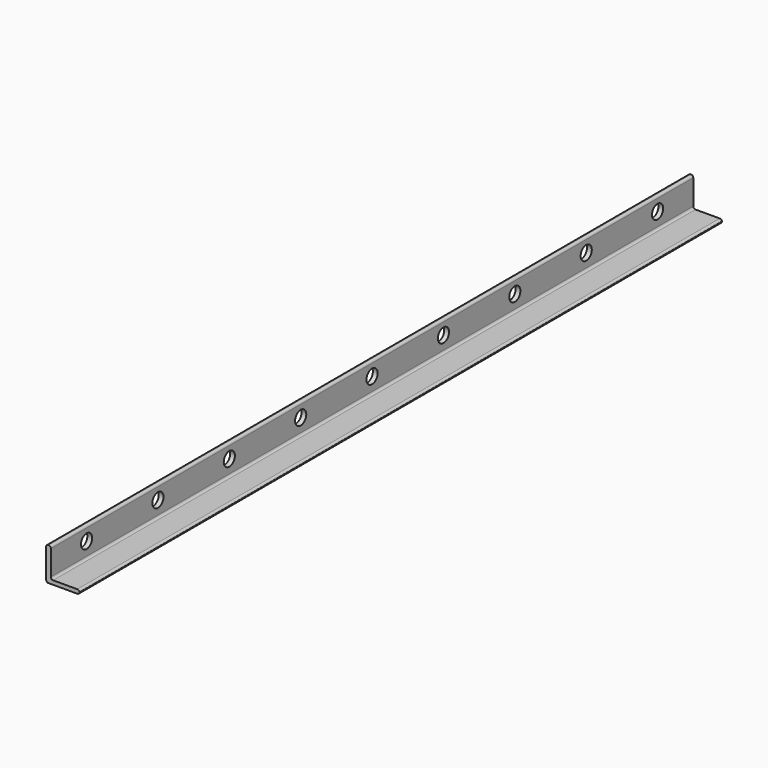
from build123d import *

# Parameters (mm, degrees)
F1_DEPTH    = 228.6
F3_D        = 7.9375
F4_T1_DEPTH = 457.2
F4_T3_DEPTH = 463.55


# Not quite as in the source:
# - a fillet or chamfer that OpenCascade refuses, or shapes differently, is made with other operations: its cross-section is extruded or revolved along the edge and cut away or added


with BuildPart() as f1:
    # F0 (on Front) → F1 (new body, symmetric)
    with BuildSketch(Plane.XZ):
        Polygon((0, 2.264165209), (0, 0), (2.7281190167, 0), (19.05, 0), (19.05, 2.264165209), (2.7281190167, 2.264165209), (2.7281190167, 19.05), (0, 19.05), align=None)
    extrude(amount=F1_DEPTH, both=True)

    # F3 (through all)
    with Locations(Plane.YZ.offset(2.7281190167)):
        with Locations((-203.2, 11.1125), (-152.4, 11.1125), (-101.6, 11.1125), (-50.8, 11.1125), (101.6, 11.1125), (50.8, 11.1125), (0, 11.1125), (152.4, 11.1125), (203.2, 11.1125)):
            Hole(F3_D / 2)

    # F4: fillet of radius 1.27 on 6 edges, made by hand

    # F4_s2 → F4_t1 (join)
    with BuildSketch(Plane.XZ.offset(-228.6)):
        with BuildLine():
            ThreePointArc((3.9981190167, 2.264165209), (3.1000934046, 2.6361395969), (2.7281190167, 3.534165209))
            Line((2.7281190167, 3.534165209), (2.7281190167, 2.264165209))
            Line((2.7281190167, 2.264165209), (3.9981190167, 2.264165209))
        make_face()
    extrude(amount=F4_T1_DEPTH)

    # F4_s4 → F4_t3 (cut)
    with BuildSketch(Plane.XZ.offset(-231.775)):
        with BuildLine():
            ThreePointArc((0, 17.78), (0.3719743879, 18.6780256121), (1.27, 19.05))
            Line((1.27, 19.05), (0, 19.05))
            Line((0, 19.05), (0, 17.78))
        make_face()
        with BuildLine():
            ThreePointArc((1.4581190167, 19.05), (2.3561446288, 18.6780256121), (2.7281190167, 17.78))
            Line((2.7281190167, 17.78), (2.7281190167, 19.05))
            Line((2.7281190167, 19.05), (1.4581190167, 19.05))
        make_face()
        with BuildLine():
            ThreePointArc((19.05, 0.994165209), (18.6780256121, 1.8921908211), (17.78, 2.264165209))
            Line((17.78, 2.264165209), (19.05, 2.264165209))
            Line((19.05, 2.264165209), (19.05, 0.994165209))
        make_face()
        with BuildLine():
            ThreePointArc((17.78, 0), (18.6780256121, 0.3719743879), (19.05, 1.27))
            Line((19.05, 1.27), (19.05, 0))
            Line((19.05, 0), (17.78, 0))
        make_face()
        with BuildLine():
            ThreePointArc((0, 1.27), (0.3719743879, 0.3719743879), (1.27, 0))
            Line((1.27, 0), (0, 0))
            Line((0, 0), (0, 1.27))
        make_face()
    extrude(amount=F4_T3_DEPTH, mode=Mode.SUBTRACT)


solid = f1.part
